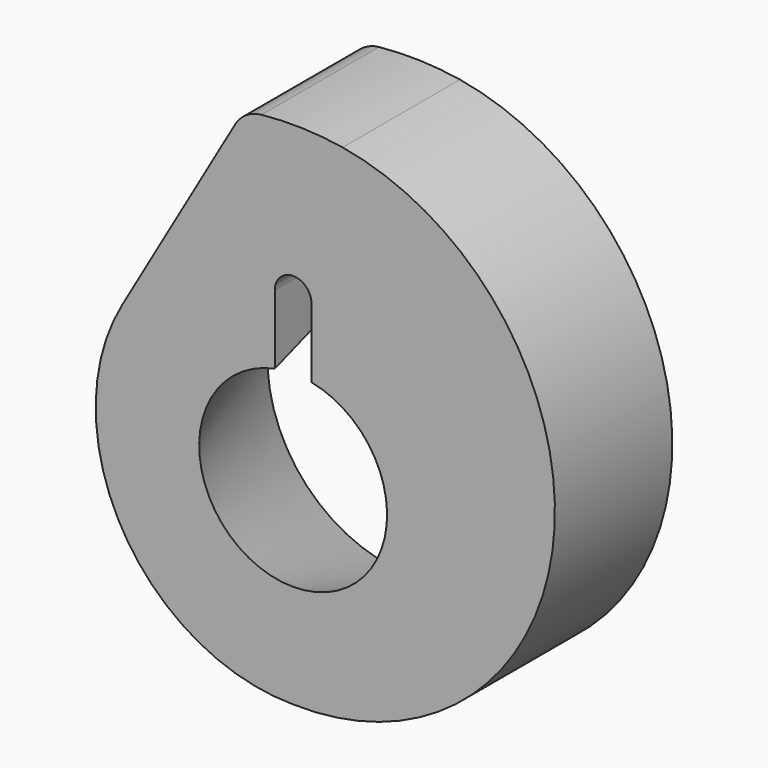
from build123d import *

# Parameters (mm, degrees)
F0_R     = 8.128
F1_DEPTH = 12.7
F5_DEPTH = 12.701


# Not quite as in the source:
# - ends of sketch curves that miss each other by under 0.0002 mm in the source are joined


with BuildPart() as f1:
    # F0 (on Front) → F1 (new body)
    with BuildSketch(Plane.XZ):
        with BuildLine():
            Line((-5.0256186, 25.460071), (-14.7940014, 8.54075))
            ThreePointArc((-14.7940014, 8.54075), (-14.7940038016, -8.5407495378), (-0.0009906, -17.0815))
            ThreePointArc((-0.0009906, -17.0815), (22.5453798959, 2.8340109101), (4.2845187845, 26.7402328229))
            ThreePointArc((4.2845187845, 26.7402328229), (0.7827449758, 27.0701370063), (-2.7322519698, 26.9433993832))
            ThreePointArc((-2.7322519698, 26.9433993832), (-4.0577155326, 26.4781440431), (-5.0256186, 25.460071))
        make_face()
        with Locations((-0.0009906, 0)):
            Circle(F0_R, mode=Mode.SUBTRACT)
    extrude(amount=-F1_DEPTH)

    # F2 (on Top) → F3 (revolve, cut)
    with BuildSketch(Plane.XY):
        Polygon((1.778, 0), (8.128, 0), (12.4623477688, 12.954), (8.128, 12.954), (1.778, 12.954), align=None)
    revolve(axis=Axis((-0.0009906, 0, 0), (0, -1, 0)), mode=Mode.SUBTRACT)

    # F4 (on face) → F5 (cut, through all)
    with BuildSketch(Plane.XZ):
        with BuildLine():
            Line((-1.5875, 13.97), (-1.5875, 3.0828800518))
            Line((-1.5875, 3.0828800518), (1.5875, 3.0828800518))
            Line((1.5875, 3.0828800518), (1.5875, 13.97))
            ThreePointArc((1.5875, 13.97), (0, 15.5575), (-1.5875, 13.97))
        make_face()
    extrude(amount=-F5_DEPTH, mode=Mode.SUBTRACT)


solid = f1.part
